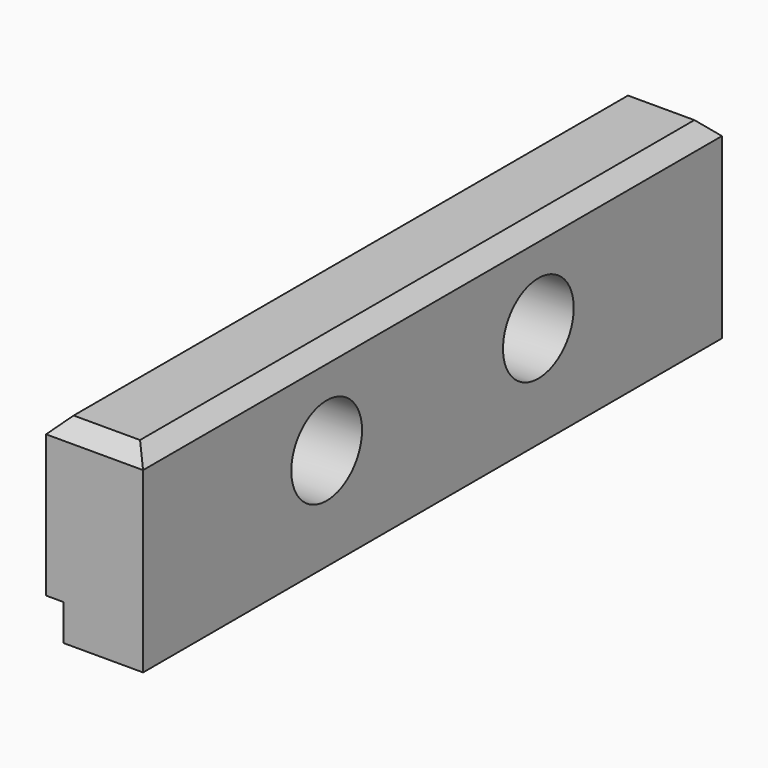
from build123d import *

# Parameters (mm, degrees)
F1_DEPTH = 240.284
F2_R     = 14.68261
F3_DEPTH = 32.216662
F4_SIZE  = 5.08
F5_T     = -2.54


with BuildPart() as f1:
    # F0 (on Front) → F1 (new body)
    with BuildSketch(Plane.XZ):
        Polygon((-47.084436, 11.595313), (-47.084436, 75.827017), (-79.300098, 75.827017), (-79.300098, 23.590051), (-73.517807, 23.590051), (-73.517807, 11.595313), align=None)
    extrude(amount=F1_DEPTH)

    # F2 (on face) → F3 (cut, through all)
    with BuildSketch(Plane.YZ.offset(-47.084436)):
        with Locations((-76.2, 45.4996)):
            Circle(F2_R)
        with Locations((-164.084, 45.4996)):
            Circle(F2_R)
    extrude(amount=-F3_DEPTH, mode=Mode.SUBTRACT)

    # F4
    f4_edges = [f1.edges().sort_by_distance(p)[0] for p in [
        (-79.300098, -120.142, 75.827017),
        (-63.192267, 0, 75.827017),
        (-47.084436, -120.142, 75.827017),
        (-63.192267, -240.284, 75.827017),
    ]]
    chamfer(f4_edges, length=F4_SIZE)

    # F5
    f5_openings = [f1.faces().sort_by_distance(p)[0] for p in [
        (-79.300098, -120.142, 47.395126),
    ]]
    offset(amount=F5_T, openings=f5_openings, kind=Kind.INTERSECTION)


solid = f1.part
